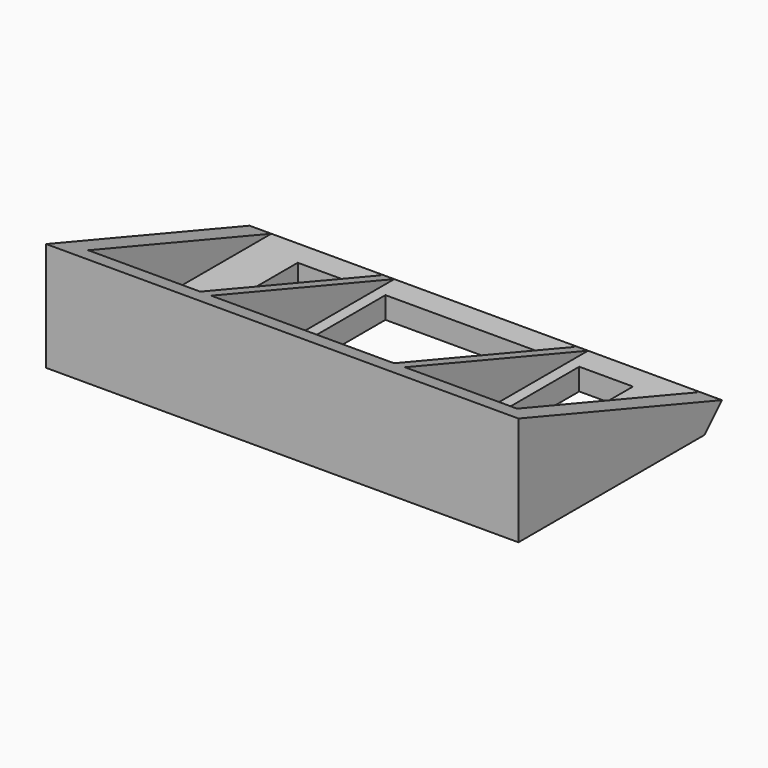
from build123d import *

# Parameters (mm, degrees)
F0_W     = 3
F0_H     = 31.5
F0_H_2   = 3.5
F0_W_2   = 1.5
F0_W_3   = 0.75
F0_H_3   = 13.2339229211
F1_DEPTH = 15
F2_DEPTH = 3
F3_SIZE  = 2.99999
F5_DEPTH = 83.7


# Not quite as in the source:
# - a fillet or chamfer is up to 0.001 mm smaller than in the source, because OpenCascade refuses the exact size


with BuildPart() as f1:
    # F0 (on Top) → F1 (new body)
    with BuildSketch(Plane.XY):
        with Locations((-31, 1.75)):
            Rectangle(F0_W, F0_H)
        with Locations((-31, -15.75)):
            Rectangle(F0_W, F0_H_2)
        with Locations((-13.3333333333, -15.75)):
            Rectangle(F0_W_2, F0_H_2)
        Polygon((-13.3333333333, 0.7660770789), (-14.0833333333, 0.7660770789), (-14.0833333333, -14), (-12.5833333333, -14), (-12.5833333333, 0.7660770789), align=None)
        with Locations((-13.7083333333, 7.3830385394)):
            Rectangle(F0_W_3, F0_H_3)
        with Locations((-12.9583333333, 7.3830385394)):
            Rectangle(F0_W_3, F0_H_3)
        with Locations((-13.7083333333, 15.75)):
            Rectangle(F0_W_3, F0_H_2)
        with Locations((-12.9583333333, 15.75)):
            Rectangle(F0_W_3, F0_H_2)
        Polygon((-12.5833333333, -14), (-12.5833333333, -17.5), (12.5833333333, -17.5), (12.5833333333, -14), (11, -14), (-11, -14), align=None)
        Polygon((-23.0666666667, -14), (-29.5, -14), (-29.5, -17.5), (-14.0833333333, -17.5), (-14.0833333333, -14), (-15.6666666667, -14), (-19.3666666667, -14), align=None)
        with Locations((13.3333333333, -15.75)):
            Rectangle(F0_W_2, F0_H_2)
        with Locations((31, -15.75)):
            Rectangle(F0_W, F0_H_2)
        Polygon((13.3333333333, 14), (12.5833333333, 14), (12.5833333333, 0.7660770789), (12.5833333333, -14), (14.0833333333, -14), (14.0833333333, 0.7660770789), (14.0833333333, 14), align=None)
        with Locations((13.7083333333, 15.75)):
            Rectangle(F0_W_3, F0_H_2)
        with Locations((12.9583333333, 15.75)):
            Rectangle(F0_W_3, F0_H_2)
        Polygon((14.0833333333, -14), (14.0833333333, -17.5), (29.5, -17.5), (29.5, -14), (23.0666666667, -14), (19.3666666667, -14), (15.6666666667, -14), align=None)
        with Locations((31, 1.75)):
            Rectangle(F0_W, F0_H)
    extrude(amount=F1_DEPTH)

    # F0 (on Top) → F2 (join)
    with BuildSketch(Plane.XY):
        Polygon((-14.0833333333, 17.5), (-29.5, 17.5), (-29.5, -14), (-23.0666666667, -14), (-23.0666666667, 14), (-19.3666666667, 14), (-15.6666666667, 14), (-14.0833333333, 14), align=None)
        Polygon((-14.0833333333, 0.7660770789), (-14.0833333333, 14), (-15.6666666667, 14), (-15.6666666667, -14), (-14.0833333333, -14), align=None)
        Polygon((-11, 14), (-12.5833333333, 14), (-12.5833333333, 0.7660770789), (-12.5833333333, -14), (-11, -14), align=None)
        Polygon((12.5833333333, 17.5), (-12.5833333333, 17.5), (-12.5833333333, 14), (-11, 14), (11, 14), (12.5833333333, 14), align=None)
        with Locations((-13.7083333333, 15.75)):
            Rectangle(F0_W_3, F0_H_2)
        with Locations((-12.9583333333, 15.75)):
            Rectangle(F0_W_3, F0_H_2)
        Polygon((29.5, 17.5), (14.0833333333, 17.5), (14.0833333333, 14), (15.6666666667, 14), (19.3666666667, 14), (23.0666666667, 14), (23.0666666667, -14), (29.5, -14), align=None)
        Polygon((12.5833333333, 0.7660770789), (12.5833333333, 14), (11, 14), (11, -14), (12.5833333333, -14), align=None)
        Polygon((15.6666666667, 14), (14.0833333333, 14), (14.0833333333, 0.7660770789), (14.0833333333, -14), (15.6666666667, -14), align=None)
    extrude(amount=F2_DEPTH)

    # F3 (size 3 in the source; OpenCascade refuses exactly that, so slightly less here)
    f3_edges = [f1.edges().sort_by_distance(p)[0] for p in [
        (0, 17.5, 0),
    ]]
    chamfer(f3_edges, length=F3_SIZE)

    # F4 (on face) → F5 (cut)
    with BuildSketch(Plane.YZ.offset(32.5)):
        Polygon((-17.5, 15), (17.5, 3), (17.5, 15), align=None)
    extrude(amount=-F5_DEPTH, mode=Mode.SUBTRACT)


solid = f1.part
